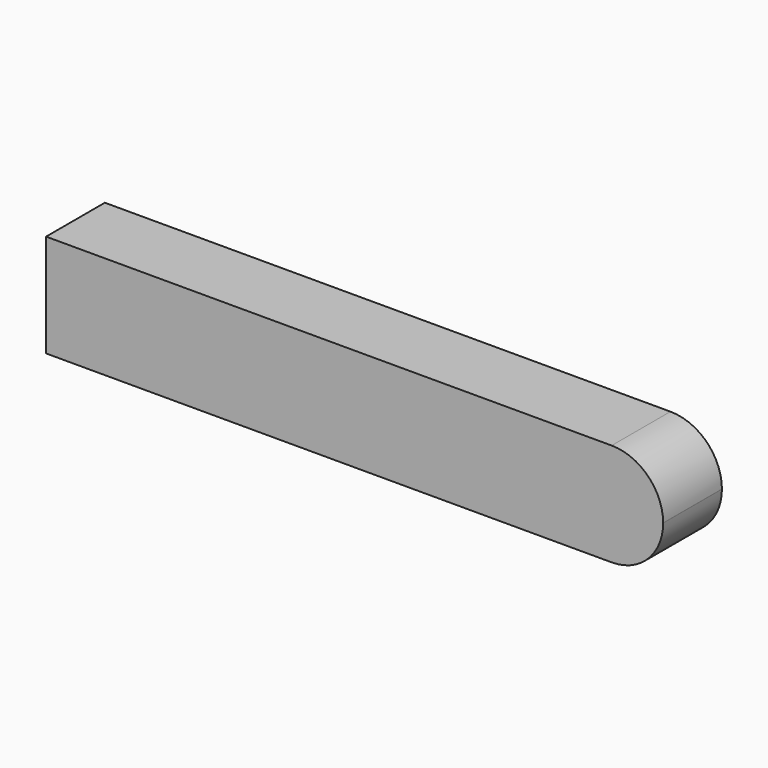
from build123d import *

# Parameters (mm, degrees)
F1_DEPTH = 15.875


# Not quite as in the source:
# - ends of sketch curves that miss each other by under 0.0002 mm in the source are joined


with BuildPart() as f1:
    # F0 (on Front) → F1 (new body)
    with BuildSketch(Plane.XZ):
        with BuildLine():
            Line((48.5642753523, 9.5875316944), (-73.6605246477, 9.5875316944))
            Line((-73.6605246477, 9.5875316944), (-73.6605246477, -12.6374683056))
            Line((-73.6605246477, -12.6374683056), (48.5642753523, -12.6374683056))
            ThreePointArc((48.5642753523, -12.6374683056), (56.4219943501, -9.3879477805), (59.689446357, -1.5376682394))
            Line((59.689446357, -1.5376682394), (59.6894753523, -1.5122683056))
            ThreePointArc((59.6894753523, -1.5122683056), (56.4219943501, 6.3380111693), (48.5642753523, 9.5875316944))
        make_face()
    extrude(amount=F1_DEPTH)


solid = f1.part
